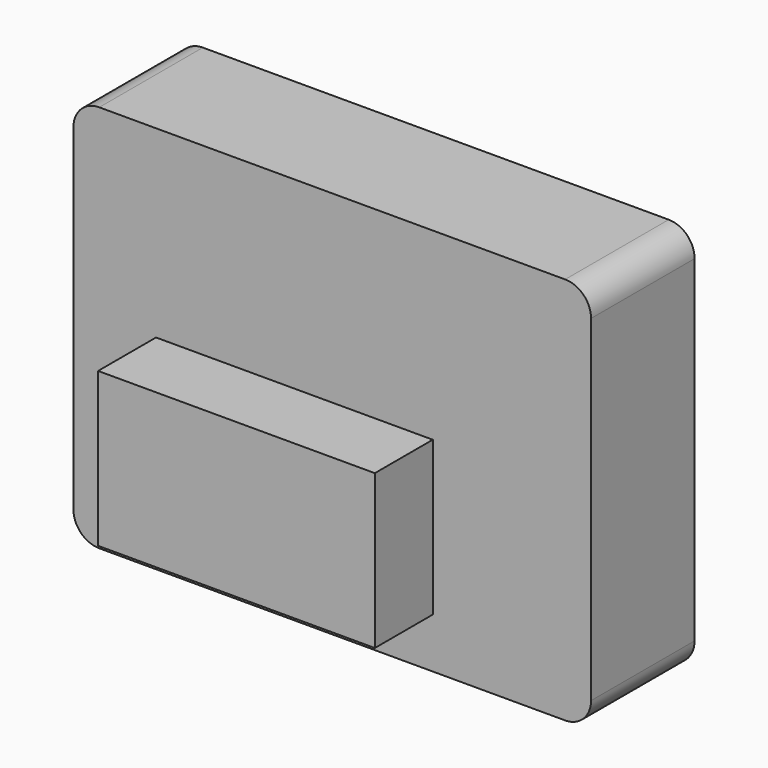
from build123d import *

# Parameters (mm, degrees)
F0_W     = 101.6
F0_H     = 76.2
F1_DEPTH = 25.4
F4_R     = 5.08
F5_W     = 54.3147437274
F5_H     = 30.2147697657
F6_DEPTH = 14.2107922584


# Not quite as in the source:
# - the program builds the solid bodies; features that only make, move or delete a surface that nothing else refers to are left out


with BuildPart() as f1:
    # F0 (on Front) → F1 (new body)
    with BuildSketch(Plane.XZ):
        with Locations((-50.8, 38.1)):
            Rectangle(F0_W, F0_H)
    extrude(amount=F1_DEPTH)

    # F4
    f4_edges = [f1.edges().sort_by_distance(p)[0] for p in [
        (-101.6, -12.7, 76.2),
        (0, -12.7, 76.2),
        (0, -12.7, 0),
        (-101.6, -12.7, 0),
    ]]
    fillet(f4_edges, radius=F4_R)

    # F5 (on face) → F6 (join)
    with BuildSketch(Plane.XZ.offset(25.4)):
        with Locations((-58.2285393029, 24.9443138018)):
            Rectangle(F5_W, F5_H)
    extrude(amount=F6_DEPTH)


solid = f1.part
